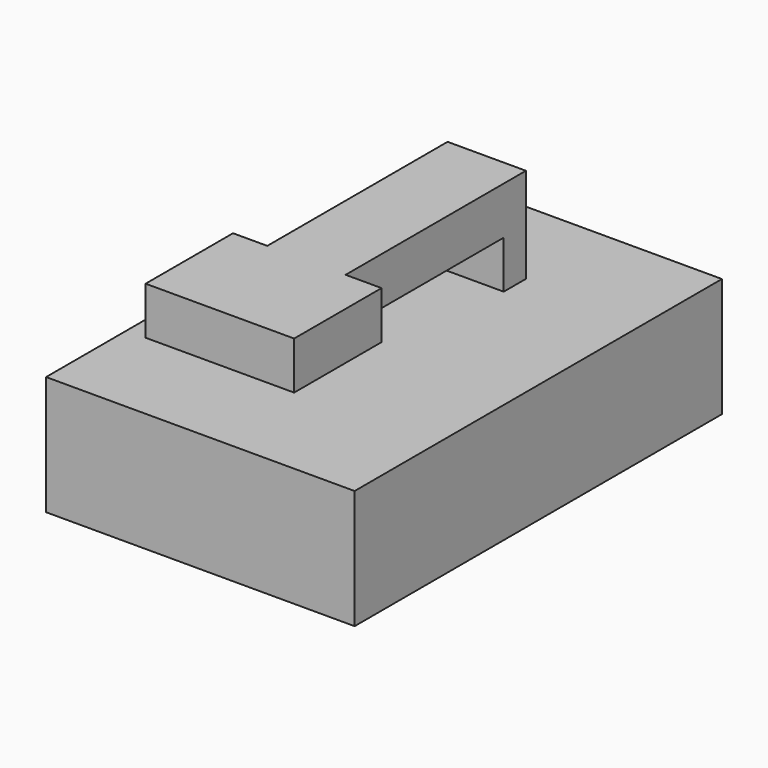
from build123d import *

# Parameters (mm, degrees)
F0_W     = 16.462284606
F0_H     = 24.4974466041
F1_DEPTH = 6.35
F3_W     = 4.1798030725
F3_H     = 1.4798403718
F4_DEPTH = 2.54
F5_W     = 4.1798030725
F5_H     = 12.0247541927
F5_H_2   = 5.8034774847
F6_DEPTH = 2.54


with BuildPart() as f1:
    # F0 (on Top) → F1 (new body)
    with BuildSketch(Plane.XY):
        with Locations((0.2442786936, 0.227171462)):
            Rectangle(F0_W, F0_H)
    extrude(amount=F1_DEPTH)


with BuildPart() as f4:
    # F3 (on face) → F4 (new body)
    with BuildSketch(Plane.XY.offset(6.35)):
        with Locations((0.0016469858, 6.6424182151)):
            Rectangle(F3_W, F3_H)
    extrude(amount=F4_DEPTH)

    # F5 (on face) → F6 (join)
    with BuildSketch(Plane.XY.offset(8.89)):
        with Locations((0.0016469858, 1.3699613046)):
            Rectangle(F5_W, F5_H)
        with Locations((0.0016469858, -7.5441545341)):
            Rectangle(F5_W, F5_H_2)
        Polygon((-2.0882545505, -10.4458932765), (-2.0882545505, -4.6424157917), (-3.9152200043, -4.6424157917), (-3.9152200043, -10.4728732258), (4.009673401, -10.4728732258), (4.009673401, -4.6424157917), (2.091548522, -4.6424157917), (2.091548522, -10.4458932765), align=None)
    extrude(amount=F6_DEPTH)


solid = Compound([f1.part, f4.part])
